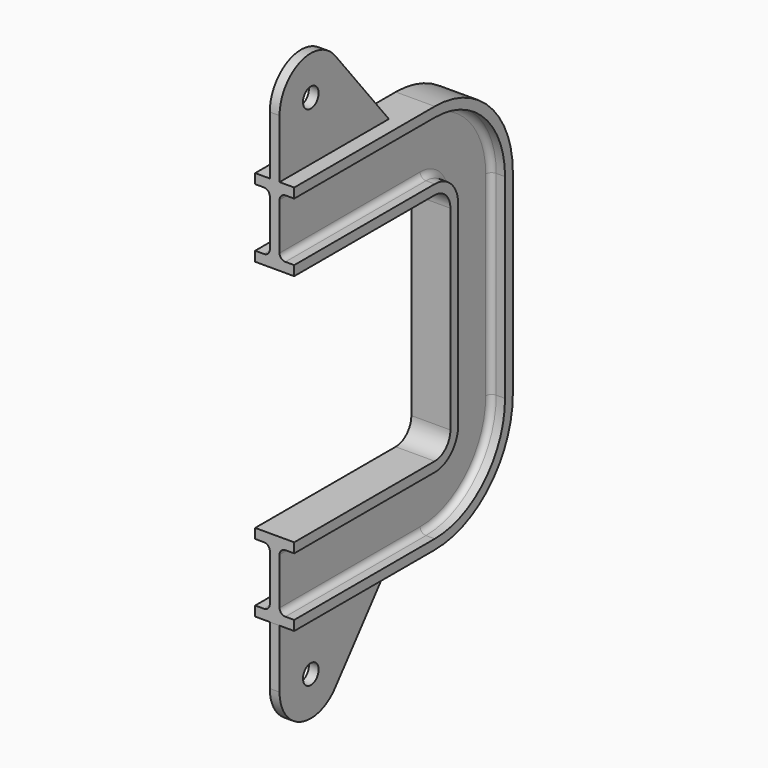
from build123d import *

# Parameters (mm, degrees)
F3_R     = 5
F4_DEPTH = 2.5


# Not quite as in the source:
# - a feature names something its author has since deleted; it is built from what else it names


with BuildPart() as f2:
    # F2: sweep along a path in F1
    with BuildLine(Plane.YZ) as f2_path:
        Line((0, -20), (90, -20))
        ThreePointArc((90, -20), (97.0710678119, -22.9289321881), (100, -30))
        Line((100, -30), (100, -80))
        Line((100, -80), (100, -130))
        ThreePointArc((100, -130), (97.0710678119, -137.0710678119), (90, -140))
        Line((90, -140), (0, -140))
    # F0 (on Front) → F2 (sweep)
    with BuildSketch(Plane.XZ):
        with BuildLine():
            Line((2.5, -12), (2.5, 0))
            Line((2.5, 0), (2.5, 12))
            ThreePointArc((2.5, 12), (3.3786796564, 14.1213203436), (5.5, 15))
            Line((5.5, 15), (10, 15))
            Line((10, 15), (10, 20))
            Line((10, 20), (0, 20))
            Line((0, 20), (-10, 20))
            Line((-10, 20), (-10, 15))
            Line((-10, 15), (-5.5, 15))
            ThreePointArc((-5.5, 15), (-3.3786796564, 14.1213203436), (-2.5, 12))
            Line((-2.5, 12), (-2.5, 0))
            Line((-2.5, 0), (-2.5, -12))
            ThreePointArc((-2.5, -12), (-3.3786796564, -14.1213203436), (-5.5, -15))
            Line((-5.5, -15), (-10, -15))
            Line((-10, -15), (-10, -20))
            Line((-10, -20), (0, -20))
            Line((0, -20), (10, -20))
            Line((10, -20), (10, -15))
            Line((10, -15), (5.5, -15))
            ThreePointArc((5.5, -15), (3.3786796564, -14.1213203436), (2.5, -12))
        make_face()
    sweep(path=f2_path.line)

    # F3 (on Right) → F4 (join, symmetric)
    with BuildSketch(Plane.YZ):
        with BuildLine():
            Line((0, 50), (0, 20))
            Line((0, 20), (70, 20))
            Line((70, 20), (35.5480451324, 62.5800752207))
            ThreePointArc((35.5480451324, 62.5800752207), (13.3277028936, 68.8541892248), (0, 50))
        make_face()
        with Locations((20, 50)):
            Circle(F3_R, mode=Mode.SUBTRACT)
        with BuildLine():
            Line((70, -180), (0, -180))
            Line((0, -180), (0, -210))
            ThreePointArc((0, -210), (13.3277028936, -228.8541892248), (35.5480451324, -222.5800752207))
            Line((35.5480451324, -222.5800752207), (70, -180))
        make_face()
        with Locations((20, -210)):
            Circle(F3_R, mode=Mode.SUBTRACT)
    extrude(amount=F4_DEPTH, both=True)


solid = f2.part
